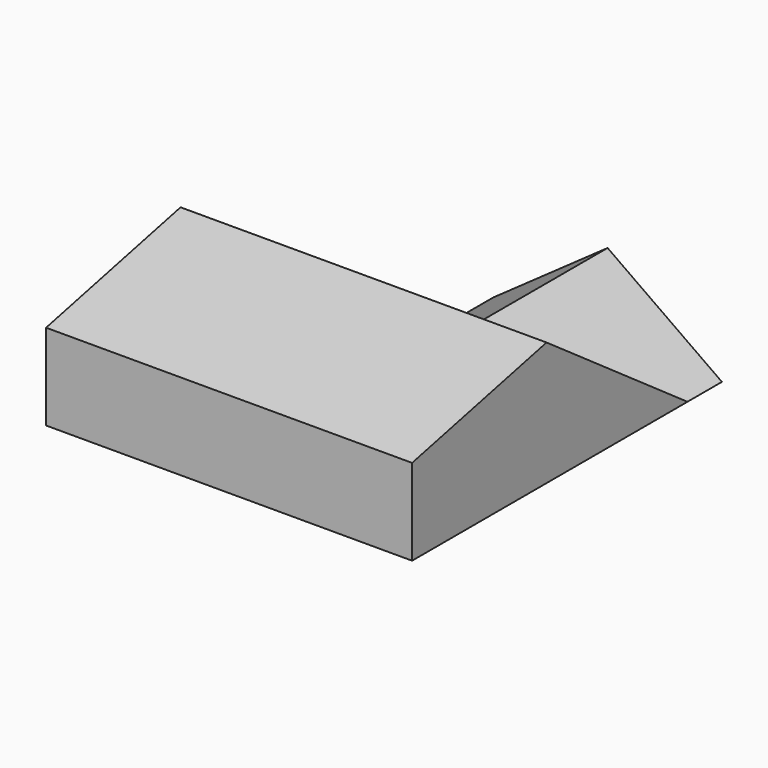
from build123d import *

# Parameters (mm, degrees)
F1_DEPTH = 10363.2
F5_DEPTH = 4572


with BuildPart() as f1:
    # F0 (on Right) → F1 (new body)
    with BuildSketch(Plane.YZ):
        Polygon((0, 2438.4), (0, 0), (9746.151653591, 0), (4758.6884747796, 3505.2), align=None)
    extrude(amount=F1_DEPTH)

    # F4 (on face) → F5 (join)
    with BuildSketch(Plane.XZ.offset(-10965.351653591)):
        Polygon((3890.2353747298, 0), (10363.2, 0), (7126.7176873649, 2286), align=None)
    extrude(amount=F5_DEPTH)


solid = f1.part
